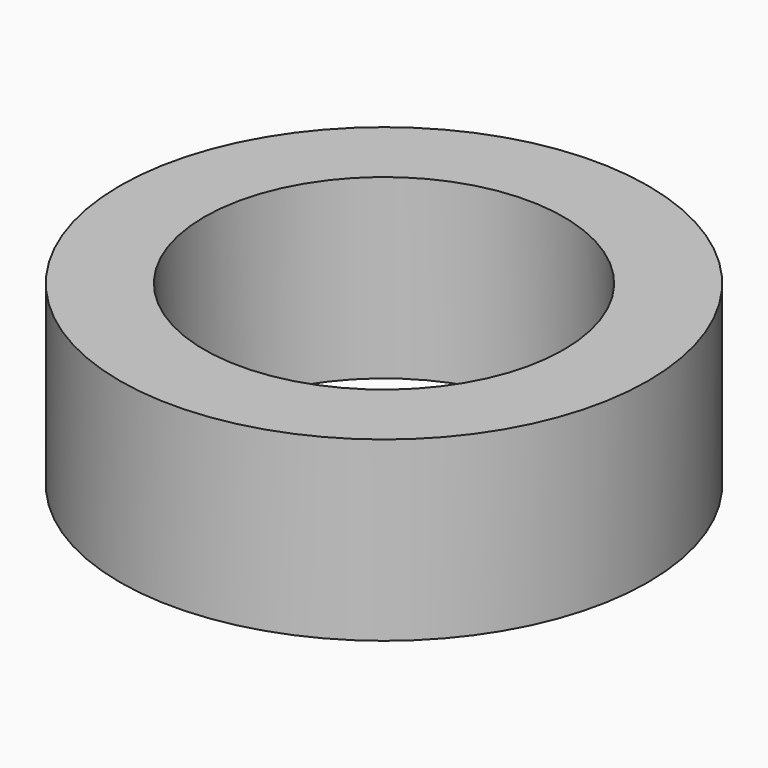
from build123d import *

# Parameters (mm, degrees)
F0_R     = 75.686993118
F1_DEPTH = 25.4
F2_DEPTH = 25.4
F7_R     = 51.508951791
F8_DEPTH = 50.801


# Not quite as in the source:
# - a feature of the source that left no trace in its solid (it failed there, or was rolled back) is left out
# - the program builds the solid bodies; features that only make, move or delete a surface that nothing else refers to are left out


with BuildPart() as f1:
    # F0 (on Top) → F1 (new body)
    with BuildSketch(Plane.XY):
        Circle(F0_R)
    extrude(amount=F1_DEPTH)

    # F2 (add): a face of the model
    f2_faces = [f1.faces().sort_by_distance(p)[0] for p in [
        (0, 0, 0),
    ]]
    extrude(f2_faces, amount=F2_DEPTH)

    # F7 (on face) → F8 (cut, through all)
    with BuildSketch(Plane(origin=(0, 0, -25.4), x_dir=(1, 0, 0), z_dir=(0, 0, -1))):
        Circle(F7_R)
    extrude(amount=-F8_DEPTH, mode=Mode.SUBTRACT)


solid = f1.part
